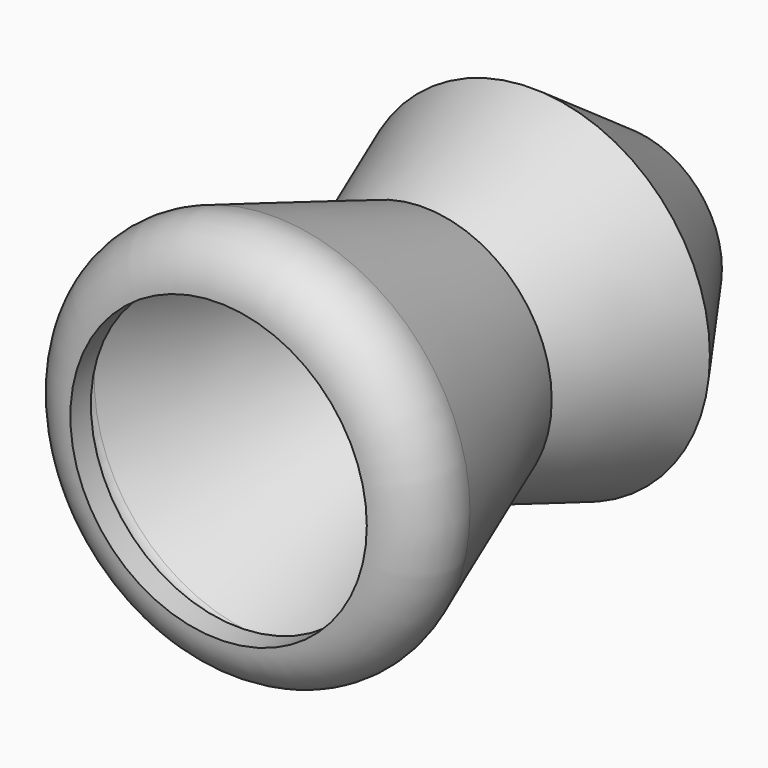
from build123d import *

# Parameters (mm, degrees)
F0_R     = 63.5
F1_DEPTH = 127
F1_TAPER = -20
F2_R     = 25.4
F3_SIZE  = 63.5
F4_T     = -12.7


# Not quite as in the source:
# - a shell that OpenCascade refuses in one call is made with other operations: the cavity is built on its own and cut out


with BuildPart() as f1:
    # F0 (on Front) → F1 (new body, symmetric)
    with BuildSketch(Plane.XZ):
        with Locations((0.2353243763, -0.2353235031)):
            Circle(F0_R)
    extrude(amount=F1_DEPTH, both=True, taper=F1_TAPER)

    # F2
    f2_edges = [f1.edges().sort_by_distance(p)[0] for p in [
        (-109.488895, -127, -0.235324),
    ]]
    fillet(f2_edges, radius=F2_R)

    # F3
    f3_edges = [f1.edges().sort_by_distance(p)[0] for p in [
        (-109.488895, 127, -0.235324),
    ]]
    chamfer(f3_edges, length=F3_SIZE)

    # F4: a shell. OpenCascade refuses it in one call, so the cavity is built on its own and cut out:
    # the body offset inwards by the wall thickness, plus a prism from it out through each open face.
    f4_core = offset(f1.part, amount=F4_T, kind=Kind.INTERSECTION, mode=Mode.PRIVATE)
    f4_exits = [f4_core.faces().sort_by_distance(p)[0] for p in [
        (0.235324, -114.3, -0.235324),
    ]]
    add(f4_core, mode=Mode.SUBTRACT)
    extrude(f4_exits, amount=-F4_T, mode=Mode.SUBTRACT)


solid = f1.part
